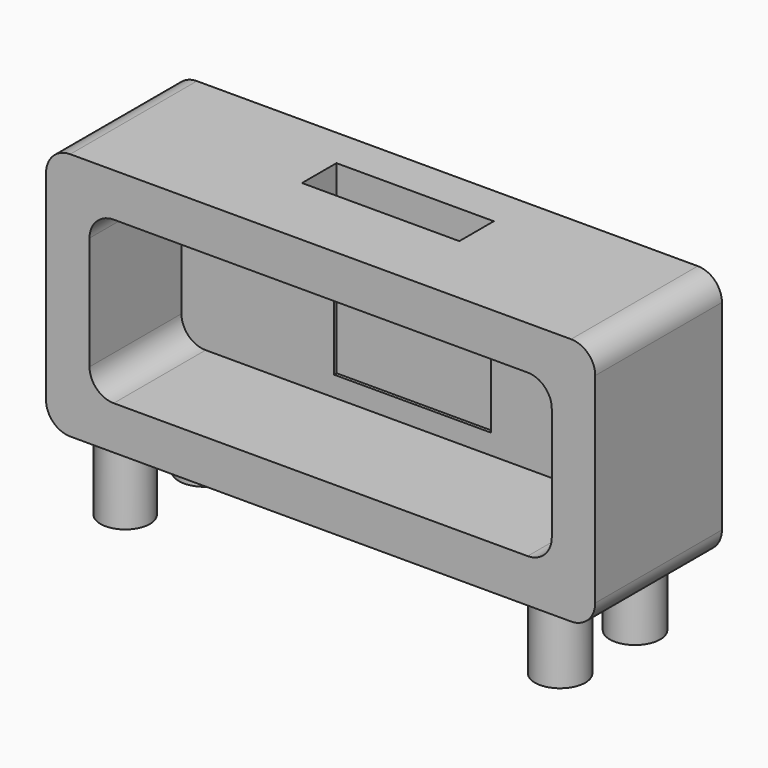
from build123d import *

# Parameters (mm, degrees)
F0_W     = 113.7392967939
F0_H     = 51.4718480408
F1_DEPTH = 32.8
F2_R     = 5
F3_T     = -9
F4_W     = 32.5862057507
F4_H     = 8.9224129915
F5_DEPTH = 38.3
F6_R     = 5
F7_R     = 5.2692974362
F7_R_2   = 5.120837474
F7_R_3   = 5.2226793455
F7_R_4   = 5.2226798643
F8_DEPTH = 15


with BuildPart() as f1:
    # F0 (on Front) → F1 (new body)
    with BuildSketch(Plane.XZ):
        Rectangle(F0_W, F0_H)
    extrude(amount=F1_DEPTH)

    # F2
    f2_edges = [f1.edges().sort_by_distance(p)[0] for p in [
        (56.869648, -16.4, 25.735924),
        (56.869648, -16.4, -25.735924),
        (-56.869648, -16.4, -25.735924),
        (-56.869648, -16.4, 25.735924),
    ]]
    fillet(f2_edges, radius=F2_R)

    # F3
    f3_openings = [f1.faces().sort_by_distance(p)[0] for p in [
        (0, -32.8, 0),
    ]]
    offset(amount=F3_T, openings=f3_openings)

    # F4 (on face) → F5 (cut)
    with BuildSketch(Plane.XY.offset(25.7359240204)):
        with Locations((0, -12.8017254174)):
            Rectangle(F4_W, F4_H)
    extrude(amount=-F5_DEPTH, mode=Mode.SUBTRACT)

    # F6
    f6_edges = [f1.edges().sort_by_distance(p)[0] for p in [
        (47.869648, -20.9, -16.735924),
        (-47.869648, -20.9, -16.735924),
        (-47.869648, -20.9, 16.735924),
        (47.869648, -20.9, 16.735924),
    ]]
    fillet(f6_edges, radius=F6_R)

    # F7 (on face) → F8 (join)
    with BuildSketch(Plane(origin=(0, 0, -25.7359240204), x_dir=(1, 0, 0), z_dir=(0, 0, -1))):
        with Locations((-45.1939664781, 6.4008627087)):
            Circle(F7_R)
        with Locations((-45.7758642733, 26.1853467673)):
            Circle(F7_R_2)
        with Locations((43.8362061977, 6.2068966217)):
            Circle(F7_R_3)
        with Locations((43.8362061977, 25.6034508348)):
            Circle(F7_R_4)
    extrude(amount=F8_DEPTH)


solid = f1.part
